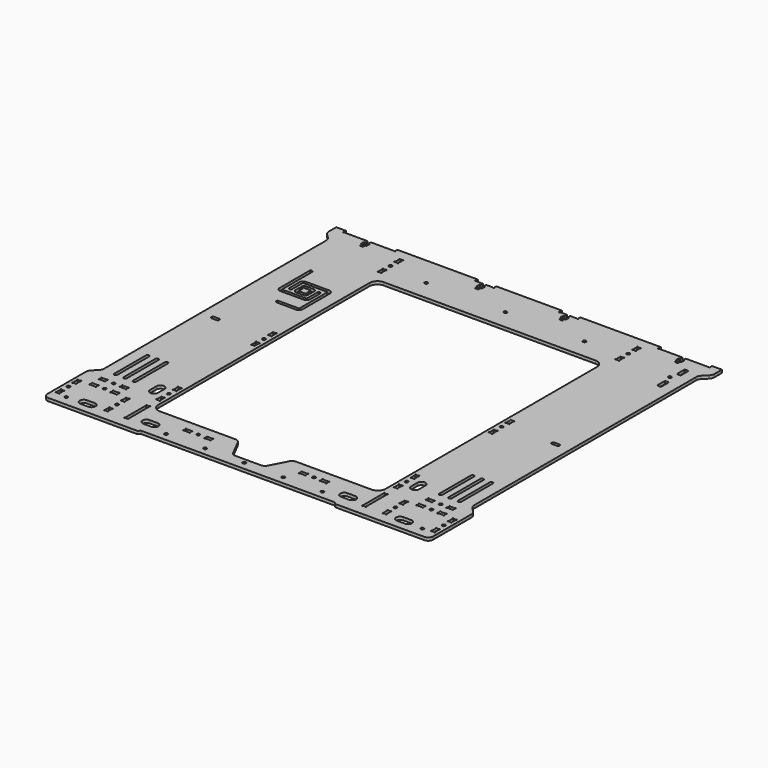
from build123d import *

# Parameters (mm, degrees)
F0_R     = 1.6
F1_DEPTH = 3


# Not quite as in the source:
# - ends of sketch curves that miss each other by under 0.0002 mm in the source are joined


with BuildPart() as f1:
    # F0 (on Top) → F1 (new body)
    with BuildSketch(Plane.XY):
        with BuildLine():
            Line((100.414611, -181.152447), (189.999995, -181.152721))
            ThreePointArc((189.999995, -181.152721), (193.5355256737, -179.6882531382), (194.99999, -176.152721))
            Line((194.99999, -176.152721), (194.99999, -127.617048))
            ThreePointArc((194.99999, -127.617048), (194.5500896571, -125.3374879994), (193.2678587346, -123.3997862741))
            Line((193.2678587346, -123.3997862741), (188.732131, -118.809631))
            ThreePointArc((188.732131, -118.809631), (187.4499003445, -116.8719290045), (187, -114.592369))
            Line((187, -114.592369), (187, 166.362005))
            ThreePointArc((187, 166.362005), (187.4567226696, 168.6581052675), (188.7573588129, 170.6046451871))
            Line((188.7573588129, 170.6046451871), (193.242641, 175.089927))
            ThreePointArc((193.242641, 175.089927), (194.5432773304, 177.0364667325), (195, 179.332567))
            Line((195, 179.332567), (195, 188.847286))
            Line((195, 188.847286), (185, 188.84728))
            Line((185, 188.84728), (185, 186.61326))
            ThreePointArc((185, 186.61326), (185.0669869604, 186.363259585), (185.2499996961, 186.1802464736))
            ThreePointArc((185.2499996961, 186.1802464736), (185.3535528736, 185.3936810924), (184.5669873396, 185.4972321961))
            ThreePointArc((184.5669873396, 185.4972321961), (184.3839752565, 185.6802441311), (184.133976, 185.747231))
            Line((184.133976, 185.747231), (160.775004, 185.747234))
            Line((160.775004, 185.747234), (160.775004, 182.747263))
            Line((160.775004, 182.747263), (162.049999, 182.747263))
            Line((162.049999, 182.747263), (162.049999, 178.747234))
            Line((162.049999, 178.747234), (160.775004, 178.747234))
            Line((160.775004, 178.747234), (160.775004, 175.747234))
            Line((160.775004, 175.747234), (157.574993, 175.747234))
            Line((157.574993, 175.747234), (157.574993, 178.747234))
            Line((157.574993, 178.747234), (156.299999, 178.747234))
            Line((156.299999, 178.747234), (156.299999, 182.747263))
            Line((156.299999, 182.747263), (157.574993, 182.747263))
            Line((157.574993, 182.747263), (157.574993, 185.747234))
            Line((157.574993, 185.747234), (134.066026, 185.74684))
            ThreePointArc((134.066026, 185.74684), (133.816025585, 185.6798530396), (133.6330124736, 185.4968403039))
            ThreePointArc((133.6330124736, 185.4968403039), (132.8464473986, 185.3932858203), (132.9499981961, 186.1798516604))
            ThreePointArc((132.9499981961, 186.1798516604), (133.1330100061, 186.362864527), (133.199997, 186.612864))
            Line((133.199997, 186.612864), (133.2, 188.846886))
            Line((133.2, 188.846886), (51.734412, 188.846886))
            Line((51.734412, 188.846886), (51.734412, 186.61287))
            ThreePointArc((51.734412, 186.61287), (51.8013990854, 186.3628693685), (51.9844121291, 186.1798562236))
            ThreePointArc((51.9844121291, 186.1798562236), (52.087966003, 185.3932912218), (51.3014003396, 185.4968421961))
            ThreePointArc((51.3014003396, 185.4968421961), (51.118387473, 185.6798540061), (50.868388, 185.746841))
            Line((50.868388, 185.746841), (44.100912, 185.74689))
            Line((44.100912, 185.74689), (44.100912, 182.74789))
            Line((44.100912, 182.74789), (45.375891, 182.747969))
            Line((45.375891, 182.747969), (45.375891, 178.747941))
            Line((45.375891, 178.747941), (44.100896, 178.747941))
            Line((44.100896, 178.747941), (44.100896, 175.747941))
            Line((44.100896, 175.747941), (40.900885, 175.747941))
            Line((40.900885, 175.747941), (40.900885, 178.747941))
            Line((40.900885, 178.747941), (39.625891, 178.747941))
            Line((39.625891, 178.747941), (39.625891, 182.747969))
            Line((39.625891, 182.747969), (40.900912, 182.74689))
            Line((40.900912, 182.74689), (40.900912, 185.74789))
            Line((40.900912, 185.74789), (34.131638, 185.746844))
            ThreePointArc((34.131638, 185.746844), (33.8816379355, 185.6798566646), (33.6986252236, 185.4968438709))
            ThreePointArc((33.6986252236, 185.4968438709), (32.9120602218, 185.393289997), (33.0156111961, 186.1798556604))
            ThreePointArc((33.0156111961, 186.1798556604), (33.1986222226, 186.362868902), (33.265609, 186.612868))
            Line((33.265609, 186.612868), (33.265612, 188.84689))
            Line((33.265612, 188.84689), (-33.265588, 188.84689))
            Line((-33.265588, 188.84689), (-33.265588, 186.61287))
            ThreePointArc((-33.265588, 186.61287), (-33.1986009146, 186.3628693685), (-33.0155878709, 186.1798562236))
            ThreePointArc((-33.0155878709, 186.1798562236), (-32.912033997, 185.3932912218), (-33.6985996604, 185.4968421961))
            ThreePointArc((-33.6985996604, 185.4968421961), (-33.881612527, 185.6798540061), (-34.131612, 185.746841))
            Line((-34.131612, 185.746841), (-40.908088, 185.74689))
            Line((-40.908088, 185.74689), (-40.908088, 182.74889))
            Line((-40.908088, 182.74889), (-39.633265, 182.748947))
            Line((-39.633265, 182.748947), (-39.633265, 178.748919))
            Line((-39.633265, 178.748919), (-40.90826, 178.748919))
            Line((-40.90826, 178.748919), (-40.90826, 175.748919))
            Line((-40.90826, 175.748919), (-44.108271, 175.748919))
            Line((-44.108271, 175.748919), (-44.108271, 178.748919))
            Line((-44.108271, 178.748919), (-45.383265, 178.748919))
            Line((-45.383265, 178.748919), (-45.383265, 182.748947))
            Line((-45.383265, 182.748947), (-44.108088, 182.74689))
            Line((-44.108088, 182.74689), (-44.108088, 185.74889))
            Line((-44.108088, 185.74889), (-50.876962, 185.746844))
            ThreePointArc((-50.876962, 185.746844), (-51.1269620645, 185.6798566646), (-51.3099747764, 185.4968438709))
            ThreePointArc((-51.3099747764, 185.4968438709), (-52.0965397782, 185.393289997), (-51.9929888039, 186.1798556604))
            ThreePointArc((-51.9929888039, 186.1798556604), (-51.8099777774, 186.362868902), (-51.742991, 186.612868))
            Line((-51.742991, 186.612868), (-51.742988, 188.846886))
            Line((-51.742988, 188.846886), (-133.2, 188.846886))
            Line((-133.2, 188.846886), (-133.2, 186.612866))
            ThreePointArc((-133.2, 186.612866), (-133.1330130396, 186.362865585), (-132.9500003039, 186.1798524736))
            ThreePointArc((-132.9500003039, 186.1798524736), (-132.8464458203, 185.3932873986), (-133.6330116604, 185.4968381961))
            ThreePointArc((-133.6330116604, 185.4968381961), (-133.816024527, 185.6798500061), (-134.066024, 185.746837))
            Line((-134.066024, 185.746837), (-157.574998, 185.747234))
            Line((-157.574998, 185.747234), (-157.574998, 182.747263))
            Line((-157.574998, 182.747263), (-156.300004, 182.747263))
            Line((-156.300004, 182.747263), (-156.300004, 178.747234))
            Line((-156.300004, 178.747234), (-157.574998, 178.747234))
            Line((-157.574998, 178.747234), (-157.574998, 175.747234))
            Line((-157.574998, 175.747234), (-160.775009, 175.747234))
            Line((-160.775009, 175.747234), (-160.775009, 178.747234))
            Line((-160.775009, 178.747234), (-162.050004, 178.747234))
            Line((-162.050004, 178.747234), (-162.050004, 182.747263))
            Line((-162.050004, 182.747263), (-160.775009, 182.747263))
            Line((-160.775009, 182.747263), (-160.775009, 185.747234))
            Line((-160.775009, 185.747234), (-184.133979, 185.747234))
            ThreePointArc((-184.133979, 185.747234), (-184.3839796315, 185.6802469146), (-184.5669927764, 185.4972338709))
            ThreePointArc((-184.5669927764, 185.4972338709), (-185.3535577782, 185.393679997), (-185.2500068039, 186.1802456604))
            ThreePointArc((-185.2500068039, 186.1802456604), (-185.0669949939, 186.363258527), (-185.000008, 186.613258))
            Line((-185.000008, 186.613258), (-185.000005, 188.84728))
            Line((-185.000005, 188.84728), (-195, 188.847286))
            Line((-195, 188.847286), (-195, 179.332567))
            ThreePointArc((-195, 179.332567), (-194.5432773304, 177.0364667325), (-193.2426411871, 175.0899268129))
            Line((-193.2426411871, 175.0899268129), (-188.757359, 170.604645))
            ThreePointArc((-188.757359, 170.604645), (-187.4567226696, 168.6581052675), (-187, 166.362005))
            Line((-187, 166.362005), (-187, -114.667433))
            ThreePointArc((-187, -114.667433), (-187.4567226696, -116.9635332675), (-188.7573588129, -118.9100731871))
            Line((-188.7573588129, -118.9100731871), (-193.242636, -123.39535))
            ThreePointArc((-193.242636, -123.39535), (-194.5432721951, -125.3418904058), (-194.999995, -127.637991))
            Line((-194.999995, -127.637991), (-194.999995, -176.152721))
            ThreePointArc((-194.999995, -176.152721), (-193.5355302491, -179.6882506633), (-190, -181.152714))
            Line((-190, -181.152714), (-100.41422, -181.152447))
            ThreePointArc((-100.41422, -181.152447), (-100.0315385085, -181.0763260938), (-99.7071167188, -180.8595542812))
            Line((-99.7071167188, -180.8595542812), (-98.292898, -179.445338))
            ThreePointArc((-98.292898, -179.445338), (-97.9684741057, -179.2285663322), (-97.585791, -179.152446))
            Line((-97.585791, -179.152446), (97.586183, -179.152446))
            ThreePointArc((97.586183, -179.152446), (97.9688657791, -179.2285661969), (98.2932887812, -179.4453382188))
            Line((98.2932887812, -179.4453382188), (99.707508, -180.859554))
            ThreePointArc((99.707508, -180.859554), (100.0319295085, -181.0763260938), (100.414611, -181.152447))
        make_face()
        with Locations((-180, -171.152714)):
            Circle(F0_R, mode=Mode.SUBTRACT)
        with BuildLine():
            Line((-190.603935, -163.652718), (-189.036068, -163.652721))
            ThreePointArc((-189.036068, -163.652721), (-188.7860679355, -163.5857336646), (-188.6030552236, -163.4027208709))
            ThreePointArc((-188.6030552236, -163.4027208709), (-187.8164902218, -163.299166997), (-187.9200411961, -164.0857326604))
            ThreePointArc((-187.9200411961, -164.0857326604), (-188.1030522226, -164.268745902), (-188.170039, -164.518745))
            Line((-188.170039, -164.518745), (-188.170039, -168.986694))
            ThreePointArc((-188.170039, -168.986694), (-188.1030520396, -169.236694415), (-187.9200393039, -169.4197075264))
            ThreePointArc((-187.9200393039, -169.4197075264), (-187.8164861264, -170.2062729076), (-188.6030516604, -170.1027218039))
            ThreePointArc((-188.6030516604, -170.1027218039), (-188.7860637435, -169.9197098689), (-189.036063, -169.852723))
            Line((-189.036063, -169.852723), (-190.603933, -169.85272))
            ThreePointArc((-190.603933, -169.85272), (-190.8539336315, -169.9197070854), (-191.0369467764, -170.1027201291))
            ThreePointArc((-191.0369467764, -170.1027201291), (-191.8235117782, -170.206274003), (-191.7199608039, -169.4197083396))
            ThreePointArc((-191.7199608039, -169.4197083396), (-191.5369489939, -169.236695473), (-191.469962, -168.986696))
            Line((-191.469962, -168.986696), (-191.469959, -164.518746))
            ThreePointArc((-191.469959, -164.518746), (-191.5369462104, -164.268746152), (-191.7199586961, -164.0857334736))
            ThreePointArc((-191.7199586961, -164.0857334736), (-191.8235131797, -163.2991683986), (-191.0369473396, -163.4027191961))
            ThreePointArc((-191.0369473396, -163.4027191961), (-190.853934473, -163.5857310061), (-190.603935, -163.652718))
        make_face(mode=Mode.SUBTRACT)
        with BuildLine():
            Line((-164.000002, -165.15272), (-156.000001, -165.15272))
            ThreePointArc((-156.000001, -165.15272), (-152.000001, -169.15272), (-156.000001, -173.15272))
            Line((-156.000001, -173.15272), (-164.000002, -173.152721))
            ThreePointArc((-164.000002, -173.152721), (-168.000002, -169.15272), (-164.000002, -165.15272))
        make_face(mode=Mode.SUBTRACT)
        with Locations((-189.820001, -156.152721)):
            Circle(F0_R, mode=Mode.SUBTRACT)
        with BuildLine():
            Line((-190.603935, -142.452719), (-189.036068, -142.452722))
            ThreePointArc((-189.036068, -142.452722), (-188.7860679355, -142.3857346646), (-188.6030552236, -142.2027218709))
            ThreePointArc((-188.6030552236, -142.2027218709), (-187.8164893986, -142.0991668203), (-187.9200409461, -142.8857330934))
            ThreePointArc((-187.9200409461, -142.8857330934), (-188.1030522226, -143.068745902), (-188.170039, -143.318745))
            Line((-188.170039, -143.318745), (-188.170039, -147.786695))
            ThreePointArc((-188.170039, -147.786695), (-188.1030517896, -148.036694848), (-187.9200393039, -148.2197075264))
            ThreePointArc((-187.9200393039, -148.2197075264), (-187.8164861264, -149.0062729076), (-188.6030516604, -148.9027218039))
            ThreePointArc((-188.6030516604, -148.9027218039), (-188.7860637435, -148.7197098689), (-189.036063, -148.652723))
            Line((-189.036063, -148.652723), (-190.603933, -148.65272))
            ThreePointArc((-190.603933, -148.65272), (-190.8539336315, -148.7197070854), (-191.0369467764, -148.9027201291))
            ThreePointArc((-191.0369467764, -148.9027201291), (-191.8235126014, -149.0062751797), (-191.7199610539, -148.2197089066))
            ThreePointArc((-191.7199610539, -148.2197089066), (-191.5369489939, -148.036696473), (-191.469962, -147.786697))
            Line((-191.469962, -147.786697), (-191.469959, -143.318747))
            ThreePointArc((-191.469959, -143.318747), (-191.5369462104, -143.068747152), (-191.7199586961, -142.8857344736))
            ThreePointArc((-191.7199586961, -142.8857344736), (-191.8235131797, -142.0991693986), (-191.0369473396, -142.2027201961))
            ThreePointArc((-191.0369473396, -142.2027201961), (-190.853934473, -142.3857320061), (-190.603935, -142.452719))
        make_face(mode=Mode.SUBTRACT)
        with BuildLine():
            Line((-179.000003, -141.936648), (-179, -140.368781))
            ThreePointArc((-179, -140.368781), (-179.0669872104, -140.118781152), (-179.2499996961, -139.9357684736))
            ThreePointArc((-179.2499996961, -139.9357684736), (-179.3535541797, -139.1492033986), (-178.5669883396, -139.2527541961))
            ThreePointArc((-178.5669883396, -139.2527541961), (-178.383975473, -139.4357660061), (-178.133976, -139.502753))
            Line((-178.133976, -139.502753), (-173.666026, -139.502753))
            ThreePointArc((-173.666026, -139.502753), (-173.416026152, -139.4357657896), (-173.2330134736, -139.2527533039))
            ThreePointArc((-173.2330134736, -139.2527533039), (-172.4464475753, -139.1491976435), (-172.5499989461, -139.9357640934))
            ThreePointArc((-172.5499989461, -139.9357640934), (-172.7330110061, -140.118776527), (-172.799998, -140.368776))
            Line((-172.799998, -140.368776), (-172.800001, -141.936647))
            ThreePointArc((-172.800001, -141.936647), (-172.7330137896, -142.186646848), (-172.5500013039, -142.3696595264))
            ThreePointArc((-172.5500013039, -142.3696595264), (-172.4464456435, -143.1562254247), (-173.2330120934, -143.0526740539))
            ThreePointArc((-173.2330120934, -143.0526740539), (-173.416024527, -142.8696619939), (-173.666024, -142.802675))
            Line((-173.666024, -142.802675), (-178.133974, -142.802672))
            ThreePointArc((-178.133974, -142.802672), (-178.383974415, -142.8696589604), (-178.5669875264, -143.0526716961))
            ThreePointArc((-178.5669875264, -143.0526716961), (-179.3535526014, -143.1562261797), (-179.2500018039, -142.3696603396))
            ThreePointArc((-179.2500018039, -142.3696603396), (-179.0669899939, -142.186647473), (-179.000003, -141.936648))
        make_face(mode=Mode.SUBTRACT)
        with Locations((-165.3, -141.152714)):
            Circle(F0_R, mode=Mode.SUBTRACT)
        with BuildLine():
            Line((-157.800003, -141.936648), (-157.8, -140.368781))
            ThreePointArc((-157.8, -140.368781), (-157.8669872104, -140.118781152), (-158.0499996961, -139.9357684736))
            ThreePointArc((-158.0499996961, -139.9357684736), (-158.1535553565, -139.1492025753), (-157.3669889066, -139.2527539461))
            ThreePointArc((-157.3669889066, -139.2527539461), (-157.183976473, -139.4357660061), (-156.933977, -139.502753))
            Line((-156.933977, -139.502753), (-152.466027, -139.502753))
            ThreePointArc((-152.466027, -139.502753), (-152.216026585, -139.4357660396), (-152.0330134736, -139.2527533039))
            ThreePointArc((-152.0330134736, -139.2527533039), (-151.2464475753, -139.1491976435), (-151.3499989461, -139.9357640934))
            ThreePointArc((-151.3499989461, -139.9357640934), (-151.5330110061, -140.118776527), (-151.599998, -140.368776))
            Line((-151.599998, -140.368776), (-151.600001, -141.936647))
            ThreePointArc((-151.600001, -141.936647), (-151.5330137896, -142.186646848), (-151.3500013039, -142.3696595264))
            ThreePointArc((-151.3500013039, -142.3696595264), (-151.2464468203, -143.1562246014), (-152.0330126604, -143.0526738039))
            ThreePointArc((-152.0330126604, -143.0526738039), (-152.216025527, -142.8696619939), (-152.466025, -142.802675))
            Line((-152.466025, -142.802675), (-156.933975, -142.802672))
            ThreePointArc((-156.933975, -142.802672), (-157.183974848, -142.8696592104), (-157.3669875264, -143.0526716961))
            ThreePointArc((-157.3669875264, -143.0526716961), (-158.1535526014, -143.1562261797), (-158.0500018039, -142.3696603396))
            ThreePointArc((-158.0500018039, -142.3696603396), (-157.8669899939, -142.186647473), (-157.800003, -141.936648))
        make_face(mode=Mode.SUBTRACT)
        with BuildLine():
            Line((-141.563935, -163.652718), (-139.996068, -163.652721))
            ThreePointArc((-139.996068, -163.652721), (-139.7460679355, -163.5857336646), (-139.5630552236, -163.4027208709))
            ThreePointArc((-139.5630552236, -163.4027208709), (-138.7764902218, -163.299166997), (-138.8800411961, -164.0857326604))
            ThreePointArc((-138.8800411961, -164.0857326604), (-139.0630522226, -164.268745902), (-139.130039, -164.518745))
            Line((-139.130039, -164.518745), (-139.130039, -168.986694))
            ThreePointArc((-139.130039, -168.986694), (-139.0630520396, -169.236694415), (-138.8800393039, -169.4197075264))
            ThreePointArc((-138.8800393039, -169.4197075264), (-138.7764861264, -170.2062729076), (-139.5630516604, -170.1027218039))
            ThreePointArc((-139.5630516604, -170.1027218039), (-139.7460637435, -169.9197098689), (-139.996063, -169.852723))
            Line((-139.996063, -169.852723), (-141.563933, -169.85272))
            ThreePointArc((-141.563933, -169.85272), (-141.8139336315, -169.9197070854), (-141.9969467764, -170.1027201291))
            ThreePointArc((-141.9969467764, -170.1027201291), (-142.7835117782, -170.206274003), (-142.6799608039, -169.4197083396))
            ThreePointArc((-142.6799608039, -169.4197083396), (-142.4969489939, -169.236695473), (-142.429962, -168.986696))
            Line((-142.429962, -168.986696), (-142.429959, -164.518746))
            ThreePointArc((-142.429959, -164.518746), (-142.4969462104, -164.268746152), (-142.6799586961, -164.0857334736))
            ThreePointArc((-142.6799586961, -164.0857334736), (-142.7835131797, -163.2991683986), (-141.9969473396, -163.4027191961))
            ThreePointArc((-141.9969473396, -163.4027191961), (-141.813934473, -163.5857310061), (-141.563935, -163.652718))
        make_face(mode=Mode.SUBTRACT)
        with BuildLine():
            Line((-104.000004, -160.752745), (-96.000003, -160.752745))
            ThreePointArc((-96.000003, -160.752745), (-92.000002, -164.752745), (-96.000003, -168.752746))
            Line((-96.000003, -168.752746), (-104.000004, -168.752746))
            ThreePointArc((-104.000004, -168.752746), (-108.000005, -164.752745), (-104.000004, -160.752745))
        make_face(mode=Mode.SUBTRACT)
        with Locations((-140.78, -156.152721)):
            Circle(F0_R, mode=Mode.SUBTRACT)
        with BuildLine():
            Line((-141.563935, -142.452719), (-139.996068, -142.452722))
            ThreePointArc((-139.996068, -142.452722), (-139.7460679355, -142.3857346646), (-139.5630552236, -142.2027218709))
            ThreePointArc((-139.5630552236, -142.2027218709), (-138.7764893986, -142.0991668203), (-138.8800409461, -142.8857330934))
            ThreePointArc((-138.8800409461, -142.8857330934), (-139.0630522226, -143.068745902), (-139.130039, -143.318745))
            Line((-139.130039, -143.318745), (-139.130039, -147.786695))
            ThreePointArc((-139.130039, -147.786695), (-139.0630517896, -148.036694848), (-138.8800393039, -148.2197075264))
            ThreePointArc((-138.8800393039, -148.2197075264), (-138.7764861264, -149.0062729076), (-139.5630516604, -148.9027218039))
            ThreePointArc((-139.5630516604, -148.9027218039), (-139.7460637435, -148.7197098689), (-139.996063, -148.652723))
            Line((-139.996063, -148.652723), (-141.563933, -148.65272))
            ThreePointArc((-141.563933, -148.65272), (-141.8139336315, -148.7197070854), (-141.9969467764, -148.9027201291))
            ThreePointArc((-141.9969467764, -148.9027201291), (-142.7835126014, -149.0062751797), (-142.6799610539, -148.2197089066))
            ThreePointArc((-142.6799610539, -148.2197089066), (-142.4969489939, -148.036696473), (-142.429962, -147.786697))
            Line((-142.429962, -147.786697), (-142.429959, -143.318747))
            ThreePointArc((-142.429959, -143.318747), (-142.4969462104, -143.068747152), (-142.6799586961, -142.8857344736))
            ThreePointArc((-142.6799586961, -142.8857344736), (-142.7835131797, -142.0991693986), (-141.9969473396, -142.2027201961))
            ThreePointArc((-141.9969473396, -142.2027201961), (-141.813934473, -142.3857320061), (-141.563935, -142.452719))
        make_face(mode=Mode.SUBTRACT)
        with BuildLine():
            Line((-120.958936, -142.452719), (-119.391069, -142.452722))
            ThreePointArc((-119.391069, -142.452722), (-119.1410695024, -142.3857344146), (-118.9580572236, -142.2027218709))
            ThreePointArc((-118.9580572236, -142.2027218709), (-118.1714913986, -142.0991668203), (-118.2750429461, -142.8857330934))
            ThreePointArc((-118.2750429461, -142.8857330934), (-118.4580542226, -143.068745902), (-118.525041, -143.318745))
            Line((-118.525041, -143.318745), (-118.525041, -168.986694))
            ThreePointArc((-118.525041, -168.986694), (-118.4580540396, -169.236694415), (-118.2750413039, -169.4197075264))
            ThreePointArc((-118.2750413039, -169.4197075264), (-118.1714858203, -170.2062736014), (-118.9580523434, -170.1027216209))
            ThreePointArc((-118.9580523434, -170.1027216209), (-119.1410647435, -169.9197098689), (-119.391064, -169.852723))
            Line((-119.391064, -169.852723), (-120.958935, -169.85272))
            ThreePointArc((-120.958935, -169.85272), (-121.2089350645, -169.9197073354), (-121.3919477764, -170.1027201291))
            ThreePointArc((-121.3919477764, -170.1027201291), (-122.1785127782, -170.206274003), (-122.0749618039, -169.4197083396))
            ThreePointArc((-122.0749618039, -169.4197083396), (-121.8919499939, -169.236695473), (-121.824963, -168.986696))
            Line((-121.824963, -168.986696), (-121.82496, -143.318747))
            ThreePointArc((-121.82496, -143.318747), (-121.8919472104, -143.068747152), (-122.0749596961, -142.8857344736))
            ThreePointArc((-122.0749596961, -142.8857344736), (-122.1785141797, -142.0991693986), (-121.3919483396, -142.2027201961))
            ThreePointArc((-121.3919483396, -142.2027201961), (-121.208935473, -142.3857320061), (-120.958936, -142.452719))
        make_face(mode=Mode.SUBTRACT)
        with BuildLine():
            Line((-179.000011, -130.291654), (-179.000008, -128.723787))
            ThreePointArc((-179.000008, -128.723787), (-179.0669952104, -128.473787152), (-179.2500076961, -128.2907744736))
            ThreePointArc((-179.2500076961, -128.2907744736), (-179.3535621797, -127.5042093986), (-178.5669963396, -127.6077601961))
            ThreePointArc((-178.5669963396, -127.6077601961), (-178.383983473, -127.7907720061), (-178.133984, -127.857759))
            Line((-178.133984, -127.857759), (-173.666034, -127.857759))
            ThreePointArc((-173.666034, -127.857759), (-173.4160345024, -127.7907714146), (-173.2330222236, -127.6077588709))
            ThreePointArc((-173.2330222236, -127.6077588709), (-172.4464563986, -127.5042038203), (-172.5500079461, -128.2907700934))
            ThreePointArc((-172.5500079461, -128.2907700934), (-172.7330192226, -128.473782902), (-172.800006, -128.723782))
            Line((-172.800006, -128.723782), (-172.800009, -130.291653))
            ThreePointArc((-172.800009, -130.291653), (-172.7330217896, -130.541652848), (-172.5500093039, -130.7246655264))
            ThreePointArc((-172.5500093039, -130.7246655264), (-172.4464538203, -131.5112316014), (-173.2330203434, -131.4076796209))
            ThreePointArc((-173.2330203434, -131.4076796209), (-173.4160327435, -131.2246678689), (-173.666032, -131.157681))
            Line((-173.666032, -131.157681), (-178.133982, -131.157678))
            ThreePointArc((-178.133982, -131.157678), (-178.3839826315, -131.2246650854), (-178.5669957764, -131.4076781291))
            ThreePointArc((-178.5669957764, -131.4076781291), (-179.3535607782, -131.511232003), (-179.2500098039, -130.7246663396))
            ThreePointArc((-179.2500098039, -130.7246663396), (-179.0669979939, -130.541653473), (-179.000011, -130.291654))
        make_face(mode=Mode.SUBTRACT)
        with Locations((-165.300008, -129.50772)):
            Circle(F0_R, mode=Mode.SUBTRACT)
        with BuildLine():
            Line((-157.800011, -130.291654), (-157.800008, -128.723787))
            ThreePointArc((-157.800008, -128.723787), (-157.8669952104, -128.473787152), (-158.0500076961, -128.2907744736))
            ThreePointArc((-158.0500076961, -128.2907744736), (-158.1535633565, -127.5042085753), (-157.3669969066, -127.6077599461))
            ThreePointArc((-157.3669969066, -127.6077599461), (-157.183984473, -127.7907720061), (-156.933985, -127.857759))
            Line((-156.933985, -127.857759), (-152.466035, -127.857759))
            ThreePointArc((-152.466035, -127.857759), (-152.2160349355, -127.7907716646), (-152.0330222236, -127.6077588709))
            ThreePointArc((-152.0330222236, -127.6077588709), (-151.2464563986, -127.5042038203), (-151.3500079461, -128.2907700934))
            ThreePointArc((-151.3500079461, -128.2907700934), (-151.5330192226, -128.473782902), (-151.600006, -128.723782))
            Line((-151.600006, -128.723782), (-151.600009, -130.291653))
            ThreePointArc((-151.600009, -130.291653), (-151.5330217896, -130.541652848), (-151.3500093039, -130.7246655264))
            ThreePointArc((-151.3500093039, -130.7246655264), (-151.2464561264, -131.5112309076), (-152.0330216604, -131.4076798039))
            ThreePointArc((-152.0330216604, -131.4076798039), (-152.2160337435, -131.2246678689), (-152.466033, -131.157681))
            Line((-152.466033, -131.157681), (-156.933983, -131.157678))
            ThreePointArc((-156.933983, -131.157678), (-157.1839830645, -131.2246653354), (-157.3669957764, -131.4076781291))
            ThreePointArc((-157.3669957764, -131.4076781291), (-158.1535607782, -131.511232003), (-158.0500098039, -130.7246663396))
            ThreePointArc((-158.0500098039, -130.7246663396), (-157.8669979939, -130.541653473), (-157.800011, -130.291654))
        make_face(mode=Mode.SUBTRACT)
        with BuildLine():
            Line((-175.4, -116.152714), (-175.4, -76.152714))
            ThreePointArc((-175.4, -76.152714), (-173.8, -74.552714), (-172.2, -76.152714))
            Line((-172.2, -76.152714), (-172.2, -116.152714))
            ThreePointArc((-172.2, -116.152714), (-173.8, -117.752714), (-175.4, -116.152714))
        make_face(mode=Mode.SUBTRACT)
        with BuildLine():
            Line((-165.9, -116.152714), (-165.9, -76.152714))
            ThreePointArc((-165.9, -76.152714), (-164.3, -74.552714), (-162.7, -76.152714))
            Line((-162.7, -76.152714), (-162.7, -116.152714))
            ThreePointArc((-162.7, -116.152714), (-164.3, -117.752714), (-165.9, -116.152714))
        make_face(mode=Mode.SUBTRACT)
        with BuildLine():
            Line((-156.4, -116.152714), (-156.4, -76.152714))
            ThreePointArc((-156.4, -76.152714), (-154.8, -74.552714), (-153.2, -76.152714))
            Line((-153.2, -76.152714), (-153.2, -116.152714))
            ThreePointArc((-153.2, -116.152714), (-154.8, -117.752714), (-156.4, -116.152714))
        make_face(mode=Mode.SUBTRACT)
        with BuildLine():
            Line((-128.000001, -112.152716), (-128.000001, -120.152716))
            ThreePointArc((-128.000001, -120.152716), (-132.0000005, -124.152716), (-136.000001, -120.152717))
            Line((-136.000001, -120.152717), (-136.000001, -112.152717))
            ThreePointArc((-136.000001, -112.152717), (-132.0000015, -108.152716), (-128.000001, -112.152716))
        make_face(mode=Mode.SUBTRACT)
        with BuildLine():
            Line((-121.824919, -128.986627), (-121.824919, -124.518677))
            ThreePointArc((-121.824919, -124.518677), (-121.8919059939, -124.268677527), (-122.0749179461, -124.0856649066))
            ThreePointArc((-122.0749179461, -124.0856649066), (-122.1784687782, -123.299098997), (-121.3919034736, -123.4026526961))
            ThreePointArc((-121.3919034736, -123.4026526961), (-121.2088910645, -123.5856656646), (-120.958891, -123.652653))
            Line((-120.958891, -123.652653), (-119.391023, -123.65265))
            ThreePointArc((-119.391023, -123.65265), (-119.1410237435, -123.5856631311), (-118.9580111566, -123.4026514869))
            ThreePointArc((-118.9580111566, -123.4026514869), (-118.1714448203, -123.2990993986), (-118.2750003121, -124.0856654594))
            ThreePointArc((-118.2750003121, -124.0856654594), (-118.4580130396, -124.268678585), (-118.525, -124.518679))
            Line((-118.525, -124.518679), (-118.524997, -128.986629))
            ThreePointArc((-118.524997, -128.986629), (-118.4580102226, -129.236628098), (-118.2749988039, -129.4196406604))
            ThreePointArc((-118.2749988039, -129.4196406604), (-118.1714473986, -130.2062071797), (-118.9580132094, -130.1026521209))
            ThreePointArc((-118.9580132094, -130.1026521209), (-119.1410255024, -129.9196395854), (-119.391025, -129.852652))
            Line((-119.391025, -129.852652), (-120.958895, -129.852655))
            ThreePointArc((-120.958895, -129.852655), (-121.208894098, -129.9196417774), (-121.3919066604, -130.1026531961))
            ThreePointArc((-121.3919066604, -130.1026531961), (-122.1784728736, -130.2062049076), (-122.0749188709, -129.4196392236))
            ThreePointArc((-122.0749188709, -129.4196392236), (-121.8919062104, -129.236626848), (-121.824919, -128.986627))
        make_face(mode=Mode.SUBTRACT)
        with Locations((-120.174958, -116.152653)):
            Circle(F0_R, mode=Mode.SUBTRACT)
        with BuildLine():
            Line((-121.824919, -107.786627), (-121.824919, -103.318678))
            ThreePointArc((-121.824919, -103.318678), (-121.8919059939, -103.068678527), (-122.0749179461, -102.8856659066))
            ThreePointArc((-122.0749179461, -102.8856659066), (-122.1784687782, -102.099099997), (-121.3919034736, -102.2026536961))
            ThreePointArc((-121.3919034736, -102.2026536961), (-121.2088910645, -102.3856666646), (-120.958891, -102.452654))
            Line((-120.958891, -102.452654), (-119.391023, -102.452651))
            ThreePointArc((-119.391023, -102.452651), (-119.1410237435, -102.3856641311), (-118.9580111566, -102.2026524869))
            ThreePointArc((-118.9580111566, -102.2026524869), (-118.1714448203, -102.0991003986), (-118.2750003121, -102.8856664594))
            ThreePointArc((-118.2750003121, -102.8856664594), (-118.4580127896, -103.068679152), (-118.525, -103.318679))
            Line((-118.525, -103.318679), (-118.524997, -107.786629))
            ThreePointArc((-118.524997, -107.786629), (-118.4580102226, -108.036628098), (-118.2749988039, -108.2196406604))
            ThreePointArc((-118.2749988039, -108.2196406604), (-118.1714482218, -109.006207003), (-118.9580135264, -108.9026533039))
            ThreePointArc((-118.9580135264, -108.9026533039), (-119.1410255024, -108.7196405854), (-119.391025, -108.652653))
            Line((-119.391025, -108.652653), (-120.958895, -108.652656))
            ThreePointArc((-120.958895, -108.652656), (-121.208894473, -108.7196429939), (-121.3919070934, -108.9026549461))
            ThreePointArc((-121.3919070934, -108.9026549461), (-122.1784731797, -109.0062056014), (-122.0749188709, -108.2196402236))
            ThreePointArc((-122.0749188709, -108.2196402236), (-121.8919059604, -108.036627415), (-121.824919, -107.786627))
        make_face(mode=Mode.SUBTRACT)
        with Locations((-79.016604, -171.152746)):
            Circle(F0_R, mode=Mode.SUBTRACT)
        with BuildLine():
            Line((-72.225046, -156.936653), (-72.225043, -155.368786))
            ThreePointArc((-72.225043, -155.368786), (-72.2920305854, -155.1187865024), (-72.4750431291, -154.9357742236))
            ThreePointArc((-72.4750431291, -154.9357742236), (-72.5785958736, -154.1492090924), (-71.7920305896, -154.2527597631))
            ThreePointArc((-71.7920305896, -154.2527597631), (-71.609018098, -154.4357712226), (-71.359019, -154.502758))
            Line((-71.359019, -154.502758), (-66.891069, -154.502758))
            ThreePointArc((-66.891069, -154.502758), (-66.641069152, -154.4357707896), (-66.4580564736, -154.2527583039))
            ThreePointArc((-66.4580564736, -154.2527583039), (-65.6714903986, -154.1492028203), (-65.7750423791, -154.9357693434))
            ThreePointArc((-65.7750423791, -154.9357693434), (-65.9580541311, -155.1187817435), (-66.025041, -155.368781))
            Line((-66.025041, -155.368781), (-66.025044, -156.936652))
            ThreePointArc((-66.025044, -156.936652), (-65.9580566646, -157.1866520645), (-65.7750438709, -157.3696647764))
            ThreePointArc((-65.7750438709, -157.3696647764), (-65.6714888203, -158.1562306014), (-66.4580550934, -158.0526790539))
            ThreePointArc((-66.4580550934, -158.0526790539), (-66.641067527, -157.8696669939), (-66.891067, -157.80268))
            Line((-66.891067, -157.80268), (-71.359017, -157.802677))
            ThreePointArc((-71.359017, -157.802677), (-71.609017415, -157.8696639604), (-71.7920305264, -158.0526766961))
            ThreePointArc((-71.7920305264, -158.0526766961), (-72.5785959076, -158.1562308736), (-72.4750440539, -157.3696649066))
            ThreePointArc((-72.4750440539, -157.3696649066), (-72.2920327774, -157.186652098), (-72.225046, -156.936653))
        make_face(mode=Mode.SUBTRACT)
        with Locations((-58.525043, -156.152719)):
            Circle(F0_R, mode=Mode.SUBTRACT)
        with Locations((-39.508604, -171.152746)):
            Circle(F0_R, mode=Mode.SUBTRACT)
        with BuildLine():
            Line((-51.025046, -156.936653), (-51.025043, -155.368786))
            ThreePointArc((-51.025043, -155.368786), (-51.0920305854, -155.1187865024), (-51.2750431291, -154.9357742236))
            ThreePointArc((-51.2750431291, -154.9357742236), (-51.3785981797, -154.1492083986), (-50.5920319066, -154.2527599461))
            ThreePointArc((-50.5920319066, -154.2527599461), (-50.409019098, -154.4357712226), (-50.15902, -154.502758))
            Line((-50.15902, -154.502758), (-45.69107, -154.502758))
            ThreePointArc((-45.69107, -154.502758), (-45.441069585, -154.4357710396), (-45.2580564736, -154.2527583039))
            ThreePointArc((-45.2580564736, -154.2527583039), (-44.4714903986, -154.1492028203), (-44.5750423791, -154.9357693434))
            ThreePointArc((-44.5750423791, -154.9357693434), (-44.7580541311, -155.1187817435), (-44.825041, -155.368781))
            Line((-44.825041, -155.368781), (-44.825044, -156.936652))
            ThreePointArc((-44.825044, -156.936652), (-44.7580566646, -157.1866520645), (-44.5750438709, -157.3696647764))
            ThreePointArc((-44.5750438709, -157.3696647764), (-44.471489997, -158.1562297782), (-45.2580556604, -158.0526788039))
            ThreePointArc((-45.2580556604, -158.0526788039), (-45.441068527, -157.8696669939), (-45.691068, -157.80268))
            Line((-45.691068, -157.80268), (-50.159018, -157.802677))
            ThreePointArc((-50.159018, -157.802677), (-50.409017848, -157.8696642104), (-50.5920305264, -158.0526766961))
            ThreePointArc((-50.5920305264, -158.0526766961), (-51.3785959076, -158.1562308736), (-51.2750440539, -157.3696649066))
            ThreePointArc((-51.2750440539, -157.3696649066), (-51.0920327774, -157.186652098), (-51.025046, -156.936653))
        make_face(mode=Mode.SUBTRACT)
        with BuildLine():
            Line((-120.958936, -3.65271), (-119.391069, -3.652713))
            ThreePointArc((-119.391069, -3.652713), (-119.1410695024, -3.5857254146), (-118.9580572236, -3.4027128709))
            ThreePointArc((-118.9580572236, -3.4027128709), (-118.1714922218, -3.299158997), (-118.2750431961, -4.0857246604))
            ThreePointArc((-118.2750431961, -4.0857246604), (-118.4580542226, -4.268737902), (-118.525041, -4.518737))
            Line((-118.525041, -4.518737), (-118.525041, -8.986687))
            ThreePointArc((-118.525041, -8.986687), (-118.4580537896, -9.236686848), (-118.2750413039, -9.4196995264))
            ThreePointArc((-118.2750413039, -9.4196995264), (-118.1714858203, -10.2062656014), (-118.9580523434, -10.1027136209))
            ThreePointArc((-118.9580523434, -10.1027136209), (-119.1410647435, -9.9197018689), (-119.391064, -9.852715))
            Line((-119.391064, -9.852715), (-120.958935, -9.852712))
            ThreePointArc((-120.958935, -9.852712), (-121.2089350645, -9.9196993354), (-121.3919477764, -10.1027121291))
            ThreePointArc((-121.3919477764, -10.1027121291), (-122.1785136014, -10.2062671797), (-122.0749620539, -9.4197009066))
            ThreePointArc((-122.0749620539, -9.4197009066), (-121.8919499939, -9.236688473), (-121.824963, -8.986689))
            Line((-121.824963, -8.986689), (-121.82496, -4.518739))
            ThreePointArc((-121.82496, -4.518739), (-121.8919469604, -4.268738585), (-122.0749596961, -4.0857254736))
            ThreePointArc((-122.0749596961, -4.0857254736), (-122.1785141797, -3.2991603986), (-121.3919483396, -3.4027111961))
            ThreePointArc((-121.3919483396, -3.4027111961), (-121.208935473, -3.5857230061), (-120.958936, -3.65271))
        make_face(mode=Mode.SUBTRACT)
        with Locations((0, -171.152714)):
            Circle(F0_R, mode=Mode.SUBTRACT)
        with Locations((39.508396, -171.152746)):
            Circle(F0_R, mode=Mode.SUBTRACT)
        with BuildLine():
            Line((44.825036, -156.936674), (44.825039, -155.368807))
            ThreePointArc((44.825039, -155.368807), (44.7580514146, -155.1188075024), (44.5750388709, -154.9357952236))
            ThreePointArc((44.5750388709, -154.9357952236), (44.4714851264, -154.1492290924), (45.2580510934, -154.2527809461))
            ThreePointArc((45.2580510934, -154.2527809461), (45.441063902, -154.4357922226), (45.691063, -154.502779))
            Line((45.691063, -154.502779), (50.159013, -154.502779))
            ThreePointArc((50.159013, -154.502779), (50.4090124976, -154.4357914146), (50.5920247764, -154.2527788709))
            ThreePointArc((50.5920247764, -154.2527788709), (51.3785906014, -154.1492238203), (51.2750390539, -154.9357900934))
            ThreePointArc((51.2750390539, -154.9357900934), (51.0920277774, -155.118802902), (51.025041, -155.368802))
            Line((51.025041, -155.368802), (51.025038, -156.936673))
            ThreePointArc((51.025038, -156.936673), (51.0920252104, -157.186672848), (51.2750376961, -157.3696855264))
            ThreePointArc((51.2750376961, -157.3696855264), (51.3785933565, -158.1562514247), (50.5920269066, -158.0527000539))
            ThreePointArc((50.5920269066, -158.0527000539), (50.409014473, -157.8696879939), (50.159015, -157.802701))
            Line((50.159015, -157.802701), (45.691065, -157.802698))
            ThreePointArc((45.691065, -157.802698), (45.4410643685, -157.8696850854), (45.2580512236, -158.0526981291))
            ThreePointArc((45.2580512236, -158.0526981291), (44.4714862218, -158.156252003), (44.5750371961, -157.3696863396))
            ThreePointArc((44.5750371961, -157.3696863396), (44.7580490061, -157.186673473), (44.825036, -156.936674))
        make_face(mode=Mode.SUBTRACT)
        with Locations((79.016396, -171.152746)):
            Circle(F0_R, mode=Mode.SUBTRACT)
        with Locations((58.525039, -156.15274)):
            Circle(F0_R, mode=Mode.SUBTRACT)
        with BuildLine():
            Line((66.025036, -156.936674), (66.025039, -155.368807))
            ThreePointArc((66.025039, -155.368807), (65.9580514146, -155.1188075024), (65.7750388709, -154.9357952236))
            ThreePointArc((65.7750388709, -154.9357952236), (65.6714838203, -154.1492293986), (66.4580500934, -154.2527809461))
            ThreePointArc((66.4580500934, -154.2527809461), (66.641062902, -154.4357922226), (66.891062, -154.502779))
            Line((66.891062, -154.502779), (71.359012, -154.502779))
            ThreePointArc((71.359012, -154.502779), (71.6090120645, -154.4357916646), (71.7920247764, -154.2527788709))
            ThreePointArc((71.7920247764, -154.2527788709), (72.5785906014, -154.1492238203), (72.4750390539, -154.9357900934))
            ThreePointArc((72.4750390539, -154.9357900934), (72.2920277774, -155.118802902), (72.225041, -155.368802))
            Line((72.225041, -155.368802), (72.225038, -156.936673))
            ThreePointArc((72.225038, -156.936673), (72.2920252104, -157.186672848), (72.4750376961, -157.3696855264))
            ThreePointArc((72.4750376961, -157.3696855264), (72.5785910503, -158.1562507309), (71.7920255896, -158.0527002369))
            ThreePointArc((71.7920255896, -158.0527002369), (71.609013473, -157.8696879939), (71.359014, -157.802701))
            Line((71.359014, -157.802701), (66.891064, -157.802698))
            ThreePointArc((66.891064, -157.802698), (66.6410639355, -157.8696853354), (66.4580512236, -158.0526981291))
            ThreePointArc((66.4580512236, -158.0526981291), (65.6714862218, -158.156252003), (65.7750371961, -157.3696863396))
            ThreePointArc((65.7750371961, -157.3696863396), (65.9580490061, -157.186673473), (66.025036, -156.936674))
        make_face(mode=Mode.SUBTRACT)
        with BuildLine():
            Line((95.999994, -160.752745), (103.999995, -160.752745))
            ThreePointArc((103.999995, -160.752745), (107.999996, -164.752745), (103.999995, -168.752746))
            Line((103.999995, -168.752746), (95.999994, -168.752746))
            ThreePointArc((95.999994, -168.752746), (91.999993, -164.752745), (95.999994, -160.752745))
        make_face(mode=Mode.SUBTRACT)
        with BuildLine():
            Line((139.130079, -168.986624), (139.130079, -164.518674))
            ThreePointArc((139.130079, -164.518674), (139.0630920061, -164.268674527), (138.8800800539, -164.0856619066))
            ThreePointArc((138.8800800539, -164.0856619066), (138.7765283986, -163.2990958203), (139.5630942094, -163.4026508791))
            ThreePointArc((139.5630942094, -163.4026508791), (139.7461069355, -163.5856636646), (139.996107, -163.652651))
            Line((139.996107, -163.652651), (141.563975, -163.652648))
            ThreePointArc((141.563975, -163.652648), (141.8139742565, -163.5856611311), (141.9969868434, -163.4026494869))
            ThreePointArc((141.9969868434, -163.4026494869), (142.7835531797, -163.2990973986), (142.6799976879, -164.0856634594))
            ThreePointArc((142.6799976879, -164.0856634594), (142.4969852104, -164.268676152), (142.429998, -164.518676))
            Line((142.429998, -164.518676), (142.430001, -168.986626))
            ThreePointArc((142.430001, -168.986626), (142.4969877774, -169.236625098), (142.6799991961, -169.4196376604))
            ThreePointArc((142.6799991961, -169.4196376604), (142.7835506014, -170.2062041797), (141.9969847906, -170.1026491209))
            ThreePointArc((141.9969847906, -170.1026491209), (141.8139724976, -169.9196365854), (141.563973, -169.852649))
            Line((141.563973, -169.852649), (139.996103, -169.852652))
            ThreePointArc((139.996103, -169.852652), (139.746103527, -169.9196389939), (139.5630909066, -170.1026509461))
            ThreePointArc((139.5630909066, -170.1026509461), (138.7765248203, -170.2062016014), (138.8800791291, -169.4196362236))
            ThreePointArc((138.8800791291, -169.4196362236), (139.0630917896, -169.236623848), (139.130079, -168.986624))
        make_face(mode=Mode.SUBTRACT)
        with BuildLine():
            Line((119.391063, -142.452719), (120.95893, -142.452722))
            ThreePointArc((120.95893, -142.452722), (121.2089300645, -142.3857346646), (121.3919427764, -142.2027218709))
            ThreePointArc((121.3919427764, -142.2027218709), (122.1785086014, -142.0991668203), (122.0749570539, -142.8857330934))
            ThreePointArc((122.0749570539, -142.8857330934), (121.8919457774, -143.068745902), (121.824959, -143.318745))
            Line((121.824959, -143.318745), (121.824959, -168.986694))
            ThreePointArc((121.824959, -168.986694), (121.8919459604, -169.236694415), (122.0749586961, -169.4197075264))
            ThreePointArc((122.0749586961, -169.4197075264), (122.1785118736, -170.2062729076), (121.3919463396, -170.1027218039))
            ThreePointArc((121.3919463396, -170.1027218039), (121.2089342565, -169.9197098689), (120.958935, -169.852723))
            Line((120.958935, -169.852723), (119.391065, -169.85272))
            ThreePointArc((119.391065, -169.85272), (119.1410643685, -169.9197070854), (118.9580512236, -170.1027201291))
            ThreePointArc((118.9580512236, -170.1027201291), (118.1714862218, -170.206274003), (118.2750371961, -169.4197083396))
            ThreePointArc((118.2750371961, -169.4197083396), (118.4580490061, -169.236695473), (118.525036, -168.986696))
            Line((118.525036, -168.986696), (118.525039, -143.318747))
            ThreePointArc((118.525039, -143.318747), (118.4580517896, -143.068747152), (118.2750393039, -142.8857344736))
            ThreePointArc((118.2750393039, -142.8857344736), (118.1714848203, -142.0991693986), (118.9580506604, -142.2027201961))
            ThreePointArc((118.9580506604, -142.2027201961), (119.141063527, -142.3857320061), (119.391063, -142.452719))
        make_face(mode=Mode.SUBTRACT)
        with Locations((140.78004, -156.15265)):
            Circle(F0_R, mode=Mode.SUBTRACT)
        with BuildLine():
            Line((139.130079, -147.786625), (139.130079, -143.318675))
            ThreePointArc((139.130079, -143.318675), (139.0630920061, -143.068675527), (138.8800800539, -142.8856629066))
            ThreePointArc((138.8800800539, -142.8856629066), (138.7765292218, -142.099096997), (139.5630945264, -142.2026506961))
            ThreePointArc((139.5630945264, -142.2026506961), (139.7461069355, -142.3856636646), (139.996107, -142.452651))
            Line((139.996107, -142.452651), (141.563975, -142.452648))
            ThreePointArc((141.563975, -142.452648), (141.8139742565, -142.3856611311), (141.9969868434, -142.2026494869))
            ThreePointArc((141.9969868434, -142.2026494869), (142.7835531797, -142.0990973986), (142.6799976879, -142.8856634594))
            ThreePointArc((142.6799976879, -142.8856634594), (142.4969849604, -143.068676585), (142.429998, -143.318677))
            Line((142.429998, -143.318677), (142.430001, -147.786626))
            ThreePointArc((142.430001, -147.786626), (142.4969877774, -148.036625098), (142.6799991961, -148.2196376604))
            ThreePointArc((142.6799991961, -148.2196376604), (142.7835497782, -149.006204003), (141.9969844736, -148.9026503039))
            ThreePointArc((141.9969844736, -148.9026503039), (141.8139724976, -148.7196375854), (141.563973, -148.65265))
            Line((141.563973, -148.65265), (139.996103, -148.652653))
            ThreePointArc((139.996103, -148.652653), (139.746103902, -148.7196397774), (139.5630913396, -148.9026511961))
            ThreePointArc((139.5630913396, -148.9026511961), (138.7765251264, -149.0062029076), (138.8800791291, -148.2196372236))
            ThreePointArc((138.8800791291, -148.2196372236), (139.0630917896, -148.036624848), (139.130079, -147.786625))
        make_face(mode=Mode.SUBTRACT)
        with BuildLine():
            Line((164.000002, -173.152721), (156.000001, -173.152721))
            ThreePointArc((156.000001, -173.152721), (152.000001, -169.15272), (156.000001, -165.15272))
            Line((156.000001, -165.15272), (164.000002, -165.15272))
            ThreePointArc((164.000002, -165.15272), (168.000002, -169.15272), (164.000002, -173.152721))
        make_face(mode=Mode.SUBTRACT)
        with Locations((180, -171.152714)):
            Circle(F0_R, mode=Mode.SUBTRACT)
        with BuildLine():
            Line((188.170079, -168.986617), (188.170079, -164.518667))
            ThreePointArc((188.170079, -164.518667), (188.1030920061, -164.268667527), (187.9200800539, -164.0856549066))
            ThreePointArc((187.9200800539, -164.0856549066), (187.8165283986, -163.2990888203), (188.6030942094, -163.4026438791))
            ThreePointArc((188.6030942094, -163.4026438791), (188.7861069355, -163.5856566646), (189.036107, -163.652644))
            Line((189.036107, -163.652644), (190.603975, -163.652641))
            ThreePointArc((190.603975, -163.652641), (190.8539742565, -163.5856541311), (191.0369868434, -163.4026424869))
            ThreePointArc((191.0369868434, -163.4026424869), (191.8235531797, -163.2990903986), (191.7199976879, -164.0856564594))
            ThreePointArc((191.7199976879, -164.0856564594), (191.5369852104, -164.268669152), (191.469998, -164.518669))
            Line((191.469998, -164.518669), (191.470001, -168.986619))
            ThreePointArc((191.470001, -168.986619), (191.5369877774, -169.236618098), (191.7199991961, -169.4196306604))
            ThreePointArc((191.7199991961, -169.4196306604), (191.8235506014, -170.2061971797), (191.0369847906, -170.1026421209))
            ThreePointArc((191.0369847906, -170.1026421209), (190.8539724976, -169.9196295854), (190.603973, -169.852642))
            Line((190.603973, -169.852642), (189.036103, -169.852645))
            ThreePointArc((189.036103, -169.852645), (188.786103527, -169.9196319939), (188.6030909066, -170.1026439461))
            ThreePointArc((188.6030909066, -170.1026439461), (187.8165248203, -170.2061946014), (187.9200791291, -169.4196292236))
            ThreePointArc((187.9200791291, -169.4196292236), (188.1030917896, -169.236616848), (188.170079, -168.986617))
        make_face(mode=Mode.SUBTRACT)
        with BuildLine():
            Line((151.599997, -141.936648), (151.6, -140.368781))
            ThreePointArc((151.6, -140.368781), (151.5330127896, -140.118781152), (151.3500003039, -139.9357684736))
            ThreePointArc((151.3500003039, -139.9357684736), (151.2464458203, -139.1492033986), (152.0330116604, -139.2527541961))
            ThreePointArc((152.0330116604, -139.2527541961), (152.216024527, -139.4357660061), (152.466024, -139.502753))
            Line((152.466024, -139.502753), (156.933974, -139.502753))
            ThreePointArc((156.933974, -139.502753), (157.183973848, -139.4357657896), (157.3669865264, -139.2527533039))
            ThreePointArc((157.3669865264, -139.2527533039), (158.1535524247, -139.1491976435), (158.0500010539, -139.9357640934))
            ThreePointArc((158.0500010539, -139.9357640934), (157.8669889939, -140.118776527), (157.800002, -140.368776))
            Line((157.800002, -140.368776), (157.799999, -141.936647))
            ThreePointArc((157.799999, -141.936647), (157.8669862104, -142.186646848), (158.0499986961, -142.3696595264))
            ThreePointArc((158.0499986961, -142.3696595264), (158.1535543565, -143.1562254247), (157.3669879066, -143.0526740539))
            ThreePointArc((157.3669879066, -143.0526740539), (157.183975473, -142.8696619939), (156.933976, -142.802675))
            Line((156.933976, -142.802675), (152.466026, -142.802672))
            ThreePointArc((152.466026, -142.802672), (152.216025585, -142.8696589604), (152.0330124736, -143.0526716961))
            ThreePointArc((152.0330124736, -143.0526716961), (151.2464473986, -143.1562261797), (151.3499981961, -142.3696603396))
            ThreePointArc((151.3499981961, -142.3696603396), (151.5330100061, -142.186647473), (151.599997, -141.936648))
        make_face(mode=Mode.SUBTRACT)
        with Locations((165.3, -141.152714)):
            Circle(F0_R, mode=Mode.SUBTRACT)
        with Locations((189.82004, -156.152643)):
            Circle(F0_R, mode=Mode.SUBTRACT)
        with BuildLine():
            Line((172.799997, -141.936648), (172.8, -140.368781))
            ThreePointArc((172.8, -140.368781), (172.7330127896, -140.118781152), (172.5500003039, -139.9357684736))
            ThreePointArc((172.5500003039, -139.9357684736), (172.4464446435, -139.1492025753), (173.2330110934, -139.2527539461))
            ThreePointArc((173.2330110934, -139.2527539461), (173.416023527, -139.4357660061), (173.666023, -139.502753))
            Line((173.666023, -139.502753), (178.133973, -139.502753))
            ThreePointArc((178.133973, -139.502753), (178.383973415, -139.4357660396), (178.5669865264, -139.2527533039))
            ThreePointArc((178.5669865264, -139.2527533039), (179.3535524247, -139.1491976435), (179.2500010539, -139.9357640934))
            ThreePointArc((179.2500010539, -139.9357640934), (179.0669889939, -140.118776527), (179.000002, -140.368776))
            Line((179.000002, -140.368776), (178.999999, -141.936647))
            ThreePointArc((178.999999, -141.936647), (179.0669862104, -142.186646848), (179.2499986961, -142.3696595264))
            ThreePointArc((179.2499986961, -142.3696595264), (179.3535531797, -143.1562246014), (178.5669873396, -143.0526738039))
            ThreePointArc((178.5669873396, -143.0526738039), (178.383974473, -142.8696619939), (178.133975, -142.802675))
            Line((178.133975, -142.802675), (173.666025, -142.802672))
            ThreePointArc((173.666025, -142.802672), (173.416025152, -142.8696592104), (173.2330124736, -143.0526716961))
            ThreePointArc((173.2330124736, -143.0526716961), (172.4464473986, -143.1562261797), (172.5499981961, -142.3696603396))
            ThreePointArc((172.5499981961, -142.3696603396), (172.7330100061, -142.186647473), (172.799997, -141.936648))
        make_face(mode=Mode.SUBTRACT)
        with BuildLine():
            Line((188.170079, -147.786618), (188.170079, -143.318668))
            ThreePointArc((188.170079, -143.318668), (188.1030920061, -143.068668527), (187.9200800539, -142.8856559066))
            ThreePointArc((187.9200800539, -142.8856559066), (187.8165292218, -142.099089997), (188.6030945264, -142.2026436961))
            ThreePointArc((188.6030945264, -142.2026436961), (188.7861069355, -142.3856566646), (189.036107, -142.452644))
            Line((189.036107, -142.452644), (190.603975, -142.452641))
            ThreePointArc((190.603975, -142.452641), (190.8539742565, -142.3856541311), (191.0369868434, -142.2026424869))
            ThreePointArc((191.0369868434, -142.2026424869), (191.8235531797, -142.0990903986), (191.7199976879, -142.8856564594))
            ThreePointArc((191.7199976879, -142.8856564594), (191.5369849604, -143.068669585), (191.469998, -143.31867))
            Line((191.469998, -143.31867), (191.470001, -147.786619))
            ThreePointArc((191.470001, -147.786619), (191.5369877774, -148.036618098), (191.7199991961, -148.2196306604))
            ThreePointArc((191.7199991961, -148.2196306604), (191.8235497782, -149.006197003), (191.0369844736, -148.9026433039))
            ThreePointArc((191.0369844736, -148.9026433039), (190.8539724976, -148.7196305854), (190.603973, -148.652643))
            Line((190.603973, -148.652643), (189.036103, -148.652646))
            ThreePointArc((189.036103, -148.652646), (188.786103527, -148.7196329939), (188.6030909066, -148.9026449461))
            ThreePointArc((188.6030909066, -148.9026449461), (187.8165248203, -149.0061956014), (187.9200791291, -148.2196302236))
            ThreePointArc((187.9200791291, -148.2196302236), (188.1030917896, -148.036617848), (188.170079, -147.786618))
        make_face(mode=Mode.SUBTRACT)
        with BuildLine():
            Line((118.52508, -128.986627), (118.52508, -124.518677))
            ThreePointArc((118.52508, -124.518677), (118.4580930061, -124.268677527), (118.2750810539, -124.0856649066))
            ThreePointArc((118.2750810539, -124.0856649066), (118.1715302218, -123.299098997), (118.9580955264, -123.4026526961))
            ThreePointArc((118.9580955264, -123.4026526961), (119.1411083685, -123.5856659146), (119.391109, -123.652653))
            Line((119.391109, -123.652653), (120.958976, -123.65265))
            ThreePointArc((120.958976, -123.65265), (121.2089752565, -123.5856631311), (121.3919878434, -123.4026514869))
            ThreePointArc((121.3919878434, -123.4026514869), (122.1785528736, -123.2991000924), (122.0749996209, -124.0856653434))
            ThreePointArc((122.0749996209, -124.0856653434), (121.8919869604, -124.268678585), (121.825, -124.518679))
            Line((121.825, -124.518679), (121.825003, -128.986629))
            ThreePointArc((121.825003, -128.986629), (121.8919897774, -129.236628098), (122.0750011961, -129.4196406604))
            ThreePointArc((122.0750011961, -129.4196406604), (122.1785526014, -130.2062071797), (121.3919867906, -130.1026521209))
            ThreePointArc((121.3919867906, -130.1026521209), (121.2089740645, -129.9196393354), (120.958974, -129.852652))
            Line((120.958974, -129.852652), (119.391104, -129.852655))
            ThreePointArc((119.391104, -129.852655), (119.141104527, -129.9196419939), (118.9580919066, -130.1026539461))
            ThreePointArc((118.9580919066, -130.1026539461), (118.1715258203, -130.2062046014), (118.2750801291, -129.4196392236))
            ThreePointArc((118.2750801291, -129.4196392236), (118.4580927896, -129.236626848), (118.52508, -128.986627))
        make_face(mode=Mode.SUBTRACT)
        with Locations((120.175041, -116.152653)):
            Circle(F0_R, mode=Mode.SUBTRACT)
        with BuildLine():
            Line((136, -112.152714), (136, -120.152714))
            ThreePointArc((136, -120.152714), (132, -124.152714), (128, -120.152714))
            Line((128, -120.152714), (128, -112.152714))
            ThreePointArc((128, -112.152714), (132, -108.152714), (136, -112.152714))
        make_face(mode=Mode.SUBTRACT)
        with BuildLine():
            Line((118.52508, -107.786627), (118.52508, -103.318678))
            ThreePointArc((118.52508, -103.318678), (118.4580930061, -103.068678527), (118.2750810539, -102.8856659066))
            ThreePointArc((118.2750810539, -102.8856659066), (118.1715302218, -102.099099997), (118.9580955264, -102.2026536961))
            ThreePointArc((118.9580955264, -102.2026536961), (119.1411083685, -102.3856669146), (119.391109, -102.452654))
            Line((119.391109, -102.452654), (120.958976, -102.452651))
            ThreePointArc((120.958976, -102.452651), (121.2089752565, -102.3856641311), (121.3919878434, -102.2026524869))
            ThreePointArc((121.3919878434, -102.2026524869), (122.1785528736, -102.0991010924), (122.0749996209, -102.8856663434))
            ThreePointArc((122.0749996209, -102.8856663434), (121.8919872104, -103.068679152), (121.825, -103.318679))
            Line((121.825, -103.318679), (121.825003, -107.786629))
            ThreePointArc((121.825003, -107.786629), (121.8919897774, -108.036628098), (122.0750011961, -108.2196406604))
            ThreePointArc((122.0750011961, -108.2196406604), (122.1785517782, -109.006207003), (121.3919864736, -108.9026533039))
            ThreePointArc((121.3919864736, -108.9026533039), (121.2089740645, -108.7196403354), (120.958974, -108.652653))
            Line((120.958974, -108.652653), (119.391104, -108.652656))
            ThreePointArc((119.391104, -108.652656), (119.141104527, -108.7196429939), (118.9580919066, -108.9026549461))
            ThreePointArc((118.9580919066, -108.9026549461), (118.1715258203, -109.0062056014), (118.2750801291, -108.2196402236))
            ThreePointArc((118.2750801291, -108.2196402236), (118.4580930396, -108.036627415), (118.52508, -107.786627))
        make_face(mode=Mode.SUBTRACT)
        with BuildLine():
            Line((152.466027, -127.857754), (156.933976, -127.857753))
            ThreePointArc((156.933976, -127.857753), (157.183975473, -127.7907660061), (157.3669880934, -127.6077540539))
            ThreePointArc((157.3669880934, -127.6077540539), (158.1535530503, -127.5042032691), (158.0499996209, -128.2907683434))
            ThreePointArc((158.0499996209, -128.2907683434), (157.8669869604, -128.473781585), (157.8, -128.723782))
            Line((157.8, -128.723782), (157.800003, -130.291649))
            ThreePointArc((157.800003, -130.291649), (157.8669897774, -130.541648098), (158.0500011961, -130.7246606604))
            ThreePointArc((158.0500011961, -130.7246606604), (158.1535517782, -131.511227003), (157.3669864736, -131.4076733039))
            ThreePointArc((157.3669864736, -131.4076733039), (157.1839744976, -131.2246605854), (156.933975, -131.157673))
            Line((156.933975, -131.157673), (152.466025, -131.157676))
            ThreePointArc((152.466025, -131.157676), (152.216025527, -131.2246629939), (152.0330129066, -131.4076749461))
            ThreePointArc((152.0330129066, -131.4076749461), (151.2464458203, -131.5112276014), (151.3500020621, -130.7246611076))
            ThreePointArc((151.3500020621, -130.7246611076), (151.5330150396, -130.541648415), (151.600002, -130.291648))
            Line((151.600002, -130.291648), (151.599998, -128.723778))
            ThreePointArc((151.599998, -128.723778), (151.5330110061, -128.473778527), (151.3499990539, -128.2907659066))
            ThreePointArc((151.3499990539, -128.2907659066), (151.2464482218, -127.504199997), (152.0330135264, -127.6077536961))
            ThreePointArc((152.0330135264, -127.6077536961), (152.2160263685, -127.7907669146), (152.466027, -127.857754))
        make_face(mode=Mode.SUBTRACT)
        with Locations((165.300001, -129.507713)):
            Circle(F0_R, mode=Mode.SUBTRACT)
        with BuildLine():
            Line((173.666026, -127.857751), (178.133976, -127.85775))
            ThreePointArc((178.133976, -127.85775), (178.383975473, -127.7907630061), (178.5669880934, -127.6077510539))
            ThreePointArc((178.5669880934, -127.6077510539), (179.3535543565, -127.5041995753), (179.2499986879, -128.2907654594))
            ThreePointArc((179.2499986879, -128.2907654594), (179.0669867439, -128.47377896), (179, -128.723779))
            Line((179, -128.723779), (179.000003, -130.291646))
            ThreePointArc((179.000003, -130.291646), (179.0669897774, -130.541645098), (179.2500011961, -130.7246576604))
            ThreePointArc((179.2500011961, -130.7246576604), (179.3535517782, -131.511224003), (178.5669864736, -131.4076703039))
            ThreePointArc((178.5669864736, -131.4076703039), (178.3839740645, -131.2246573354), (178.133974, -131.15767))
            Line((178.133974, -131.15767), (173.666025, -131.157673))
            ThreePointArc((173.666025, -131.157673), (173.416025527, -131.2246599939), (173.2330129066, -131.4076719461))
            ThreePointArc((173.2330129066, -131.4076719461), (172.446445997, -131.5112237782), (172.5500008791, -130.7246577906))
            ThreePointArc((172.5500008791, -130.7246577906), (172.7330140396, -130.541645415), (172.800001, -130.291645))
            Line((172.800001, -130.291645), (172.799998, -128.723775))
            ThreePointArc((172.799998, -128.723775), (172.7330110061, -128.473775527), (172.5499990539, -128.2907629066))
            ThreePointArc((172.5499990539, -128.2907629066), (172.4464482218, -127.504196997), (173.2330135264, -127.6077506961))
            ThreePointArc((173.2330135264, -127.6077506961), (173.4160259355, -127.7907636646), (173.666026, -127.857751))
        make_face(mode=Mode.SUBTRACT)
        with BuildLine():
            Line((153.2, -116.152714), (153.2, -76.152714))
            ThreePointArc((153.2, -76.152714), (154.8, -74.552714), (156.4, -76.152714))
            Line((156.4, -76.152714), (156.4, -116.152714))
            ThreePointArc((156.4, -116.152714), (154.8, -117.752714), (153.2, -116.152714))
        make_face(mode=Mode.SUBTRACT)
        with BuildLine():
            Line((162.7, -116.152714), (162.7, -76.152714))
            ThreePointArc((162.7, -76.152714), (164.3, -74.552714), (165.9, -76.152714))
            Line((165.9, -76.152714), (165.9, -116.152714))
            ThreePointArc((165.9, -116.152714), (164.3, -117.752714), (162.7, -116.152714))
        make_face(mode=Mode.SUBTRACT)
        with BuildLine():
            Line((172.2, -116.152714), (172.2, -76.152714))
            ThreePointArc((172.2, -76.152714), (173.8, -74.552714), (175.4, -76.152714))
            Line((175.4, -76.152714), (175.4, -116.152714))
            ThreePointArc((175.4, -116.152714), (173.8, -117.752714), (172.2, -116.152714))
        make_face(mode=Mode.SUBTRACT)
        with BuildLine():
            Line((-107.000003, 138.847268), (106.999998, 138.847268))
            ThreePointArc((106.999998, 138.847268), (112.6571138976, 136.5042574266), (115.000396, 130.847254))
            Line((115.000396, 130.847254), (115.000396, -136.047446))
            ThreePointArc((115.000396, -136.047446), (112.6504717432, -141.6918905878), (107.000396, -144.028243))
            Line((107.000396, -144.028243), (30.547066, -144.028446))
            ThreePointArc((30.547066, -144.028446), (27.9493535127, -144.7562229448), (26.1078631284, -146.7276900666))
            Line((26.1078631284, -146.7276900666), (17.439203, -163.45347))
            ThreePointArc((17.439203, -163.45347), (15.5977124873, -165.4249370552), (13, -166.152714))
            Line((13, -166.152714), (-13, -166.152714))
            ThreePointArc((-13, -166.152714), (-15.6046304038, -165.4207229573), (-17.4466343575, -163.4390741838))
            Line((-17.4466343575, -163.4390741838), (-26.031853, -146.742086))
            ThreePointArc((-26.031853, -146.742086), (-27.8738565962, -144.7604370427), (-30.478487, -144.028446))
            Line((-30.478487, -144.028446), (-106.999607, -144.028187))
            ThreePointArc((-106.999607, -144.028187), (-112.6499200341, -141.6919949066), (-115.0000048181, -136.047446002))
            Line((-115.0000048181, -136.047446002), (-115.000004, 130.847254))
            ThreePointArc((-115.000004, 130.847254), (-112.6568660675, 136.5041208751), (-107.000003, 138.847268))
        make_face(mode=Mode.SUBTRACT)
        with BuildLine():
            Line((119.391064, -3.65271), (120.958932, -3.652713))
            ThreePointArc((120.958932, -3.652713), (121.2089314976, -3.5857254146), (121.3919437764, -3.4027128709))
            ThreePointArc((121.3919437764, -3.4027128709), (122.1785087782, -3.299158997), (122.0749578039, -4.0857246604))
            ThreePointArc((122.0749578039, -4.0857246604), (121.8919467774, -4.268737902), (121.82496, -4.518737))
            Line((121.82496, -4.518737), (121.82496, -8.986687))
            ThreePointArc((121.82496, -8.986687), (121.8919472104, -9.236686848), (122.0749596961, -9.4196995264))
            ThreePointArc((122.0749596961, -9.4196995264), (122.1785128736, -10.2062649076), (121.3919473396, -10.1027138039))
            ThreePointArc((121.3919473396, -10.1027138039), (121.2089352565, -9.9197018689), (120.958936, -9.852715))
            Line((120.958936, -9.852715), (119.391066, -9.852712))
            ThreePointArc((119.391066, -9.852712), (119.1410659355, -9.9196993354), (118.9580532236, -10.1027121291))
            ThreePointArc((118.9580532236, -10.1027121291), (118.1714873986, -10.2062671797), (118.2750389461, -9.4197009066))
            ThreePointArc((118.2750389461, -9.4197009066), (118.4580510061, -9.236688473), (118.525038, -8.986689))
            Line((118.525038, -8.986689), (118.525041, -4.518739))
            ThreePointArc((118.525041, -4.518739), (118.4580540396, -4.268738585), (118.2750413039, -4.0857254736))
            ThreePointArc((118.2750413039, -4.0857254736), (118.1714856435, -3.2991595753), (118.9580520934, -3.4027109461))
            ThreePointArc((118.9580520934, -3.4027109461), (119.141064527, -3.5857230061), (119.391064, -3.65271))
        make_face(mode=Mode.SUBTRACT)
        with BuildLine():
            Line((-169.500003, 5.747283), (-174.500003, 5.747283))
            ThreePointArc((-174.500003, 5.747283), (-176.100003, 7.347283), (-174.500003, 8.947283))
            Line((-174.500003, 8.947283), (-169.500003, 8.947283))
            ThreePointArc((-169.500003, 8.947283), (-167.900003, 7.347283), (-169.500003, 5.747283))
        make_face(mode=Mode.SUBTRACT)
        with Locations((-120.175002, 3.847287)):
            Circle(F0_R, mode=Mode.SUBTRACT)
        with BuildLine():
            Line((-120.958936, 17.547289), (-119.391069, 17.547286))
            ThreePointArc((-119.391069, 17.547286), (-119.1410695024, 17.6142735854), (-118.9580572236, 17.7972861291))
            ThreePointArc((-118.9580572236, 17.7972861291), (-118.1714922218, 17.900840003), (-118.2750431961, 17.1142743396))
            ThreePointArc((-118.2750431961, 17.1142743396), (-118.4580542226, 16.931261098), (-118.525041, 16.681262))
            Line((-118.525041, 16.681262), (-118.525041, 12.213313))
            ThreePointArc((-118.525041, 12.213313), (-118.4580540396, 11.963312585), (-118.2750413039, 11.7802994736))
            ThreePointArc((-118.2750413039, 11.7802994736), (-118.1714858203, 10.9937333986), (-118.9580523434, 11.0972853791))
            ThreePointArc((-118.9580523434, 11.0972853791), (-119.1410647435, 11.2802971311), (-119.391064, 11.347284))
            Line((-119.391064, 11.347284), (-120.958935, 11.347287))
            ThreePointArc((-120.958935, 11.347287), (-121.2089350645, 11.2802996646), (-121.3919477764, 11.0972868709))
            ThreePointArc((-121.3919477764, 11.0972868709), (-122.1785127782, 10.993732997), (-122.0749618039, 11.7802986604))
            ThreePointArc((-122.0749618039, 11.7802986604), (-121.8919499939, 11.963311527), (-121.824963, 12.213311))
            Line((-121.824963, 12.213311), (-121.82496, 16.681261))
            ThreePointArc((-121.82496, 16.681261), (-121.8919472104, 16.931260848), (-122.0749596961, 17.1142735264))
            ThreePointArc((-122.0749596961, 17.1142735264), (-122.1785141797, 17.9008386014), (-121.3919483396, 17.7972878039))
            ThreePointArc((-121.3919483396, 17.7972878039), (-121.208935473, 17.6142759939), (-120.958936, 17.547289))
        make_face(mode=Mode.SUBTRACT)
        with BuildLine():
            Line((-149, 84.980036), (-140, 84.980036))
            ThreePointArc((-140, 84.980036), (-140.8786796564, 82.8587156564), (-143, 81.980036))
            Line((-143, 81.980036), (-150, 81.980036))
            ThreePointArc((-150, 81.980036), (-152.1213203436, 82.8587156564), (-153, 84.980036))
            Line((-153, 84.980036), (-153, 89.980036))
            Line((-153, 89.980036), (-150, 89.980036))
            Line((-150, 89.980036), (-150, 85.980036))
            ThreePointArc((-150, 85.980036), (-149.7071067812, 85.2729292188), (-149, 84.980036))
        make_face(mode=Mode.SUBTRACT)
        with BuildLine():
            Line((-144, 91.980036), (-153, 91.980036))
            ThreePointArc((-153, 91.980036), (-152.1213203436, 94.1013563436), (-150, 94.980036))
            Line((-150, 94.980036), (-143, 94.980036))
            ThreePointArc((-143, 94.980036), (-140.8786796564, 94.1013563436), (-140, 91.980036))
            Line((-140, 91.980036), (-140, 86.980036))
            Line((-140, 86.980036), (-143, 86.980036))
            Line((-143, 86.980036), (-143, 90.980036))
            ThreePointArc((-143, 90.980036), (-143.2928932188, 91.6871427812), (-144, 91.980036))
        make_face(mode=Mode.SUBTRACT)
        with BuildLine():
            Line((-159, 84.980036), (-159, 96.980036))
            ThreePointArc((-159, 96.980036), (-157.8284271247, 99.8084631247), (-155, 100.980036))
            Line((-155, 100.980036), (-132, 100.980036))
            ThreePointArc((-132, 100.980036), (-129.1715728753, 99.8084631247), (-128, 96.980036))
            Line((-128, 96.980036), (-128, 62.980036))
            ThreePointArc((-128, 62.980036), (-129.1715728753, 60.1516088753), (-132, 58.980036))
            Line((-132, 58.980036), (-151, 58.980036))
            ThreePointArc((-151, 58.980036), (-152.4142135624, 59.5658224376), (-153, 60.980036))
            Line((-153, 60.980036), (-153, 61.980036))
            Line((-153, 61.980036), (-132, 61.980036))
            ThreePointArc((-132, 61.980036), (-131.2928932188, 62.2729292188), (-131, 62.980036))
            Line((-131, 62.980036), (-131, 96.980036))
            ThreePointArc((-131, 96.980036), (-131.2928932188, 97.6871427812), (-132, 97.980036))
            Line((-132, 97.980036), (-155, 97.980036))
            ThreePointArc((-155, 97.980036), (-155.7071067812, 97.6871427812), (-156, 96.980036))
            Line((-156, 96.980036), (-156, 82.980036))
            Line((-156, 82.980036), (-157, 82.980036))
            ThreePointArc((-157, 82.980036), (-158.4142135624, 83.5658224376), (-159, 84.980036))
        make_face(mode=Mode.SUBTRACT)
        with BuildLine():
            Line((-138, 75.980036), (-161, 75.980036))
            ThreePointArc((-161, 75.980036), (-163.8284271247, 77.1516088753), (-165, 79.980036))
            Line((-165, 79.980036), (-165, 118.847286))
            Line((-165, 118.847286), (-164, 118.847286))
            ThreePointArc((-164, 118.847286), (-162.5857864376, 118.2614995624), (-162, 116.847286))
            Line((-162, 116.847286), (-162, 79.980036))
            ThreePointArc((-162, 79.980036), (-161.7071067812, 79.2729292188), (-161, 78.980036))
            Line((-161, 78.980036), (-138, 78.980036))
            ThreePointArc((-138, 78.980036), (-137.2928932188, 79.2729292188), (-137, 79.980036))
            Line((-137, 79.980036), (-137, 93.980036))
            Line((-137, 93.980036), (-136, 93.980036))
            ThreePointArc((-136, 93.980036), (-134.5857864376, 93.3942495624), (-134, 91.980036))
            Line((-134, 91.980036), (-134, 79.980036))
            ThreePointArc((-134, 79.980036), (-135.1715728753, 77.1516088753), (-138, 75.980036))
        make_face(mode=Mode.SUBTRACT)
        with BuildLine():
            Line((-120.958936, 156.347286), (-119.391069, 156.347283))
            ThreePointArc((-119.391069, 156.347283), (-119.1410695024, 156.4142705854), (-118.9580572236, 156.5972831291))
            ThreePointArc((-118.9580572236, 156.5972831291), (-118.1714922218, 156.700837003), (-118.2750431961, 155.9142713396))
            ThreePointArc((-118.2750431961, 155.9142713396), (-118.4580542226, 155.731258098), (-118.525041, 155.481259))
            Line((-118.525041, 155.481259), (-118.525041, 151.01331))
            ThreePointArc((-118.525041, 151.01331), (-118.4580540396, 150.763309585), (-118.2750413039, 150.5802964736))
            ThreePointArc((-118.2750413039, 150.5802964736), (-118.1714858203, 149.7937303986), (-118.9580523434, 149.8972823791))
            ThreePointArc((-118.9580523434, 149.8972823791), (-119.1410647435, 150.0802941311), (-119.391064, 150.147281))
            Line((-119.391064, 150.147281), (-120.958935, 150.147284))
            ThreePointArc((-120.958935, 150.147284), (-121.2089350645, 150.0802966646), (-121.3919477764, 149.8972838709))
            ThreePointArc((-121.3919477764, 149.8972838709), (-122.1785127782, 149.793729997), (-122.0749618039, 150.5802956604))
            ThreePointArc((-122.0749618039, 150.5802956604), (-121.8919499939, 150.763308527), (-121.824963, 151.013308))
            Line((-121.824963, 151.013308), (-121.82496, 155.481258))
            ThreePointArc((-121.82496, 155.481258), (-121.8919472104, 155.731257848), (-122.0749596961, 155.9142705264))
            ThreePointArc((-122.0749596961, 155.9142705264), (-122.1785141797, 156.7008356014), (-121.3919483396, 156.5972848039))
            ThreePointArc((-121.3919483396, 156.5972848039), (-121.208935473, 156.4142729939), (-120.958936, 156.347286))
        make_face(mode=Mode.SUBTRACT)
        with Locations((-120.175002, 163.847283)):
            Circle(F0_R, mode=Mode.SUBTRACT)
        with BuildLine():
            Line((-120.958936, 177.547285), (-119.391069, 177.547282))
            ThreePointArc((-119.391069, 177.547282), (-119.1410695024, 177.6142695854), (-118.9580572236, 177.7972821291))
            ThreePointArc((-118.9580572236, 177.7972821291), (-118.1714913986, 177.9008371797), (-118.2750429461, 177.1142709066))
            ThreePointArc((-118.2750429461, 177.1142709066), (-118.4580542226, 176.931258098), (-118.525041, 176.681259))
            Line((-118.525041, 176.681259), (-118.525041, 172.213309))
            ThreePointArc((-118.525041, 172.213309), (-118.4580537896, 171.963309152), (-118.2750413039, 171.7802964736))
            ThreePointArc((-118.2750413039, 171.7802964736), (-118.1714858203, 170.9937303986), (-118.9580523434, 171.0972823791))
            ThreePointArc((-118.9580523434, 171.0972823791), (-119.1410647435, 171.2802941311), (-119.391064, 171.347281))
            Line((-119.391064, 171.347281), (-120.958935, 171.347284))
            ThreePointArc((-120.958935, 171.347284), (-121.2089350645, 171.2802966646), (-121.3919477764, 171.0972838709))
            ThreePointArc((-121.3919477764, 171.0972838709), (-122.1785136014, 170.9937288203), (-122.0749620539, 171.7802950934))
            ThreePointArc((-122.0749620539, 171.7802950934), (-121.8919499939, 171.963307527), (-121.824963, 172.213307))
            Line((-121.824963, 172.213307), (-121.82496, 176.681257))
            ThreePointArc((-121.82496, 176.681257), (-121.8919472104, 176.931256848), (-122.0749596961, 177.1142695264))
            ThreePointArc((-122.0749596961, 177.1142695264), (-122.1785141797, 177.9008346014), (-121.3919483396, 177.7972838039))
            ThreePointArc((-121.3919483396, 177.7972838039), (-121.208935473, 177.6142719939), (-120.958936, 177.547285))
        make_face(mode=Mode.SUBTRACT)
        with Locations((-80, 158.847286)):
            Circle(F0_R, mode=Mode.SUBTRACT)
        with Locations((120.174999, 3.847287)):
            Circle(F0_R, mode=Mode.SUBTRACT)
        with BuildLine():
            Line((119.391064, 17.547289), (120.958932, 17.547286))
            ThreePointArc((120.958932, 17.547286), (121.2089314976, 17.6142735854), (121.3919437764, 17.7972861291))
            ThreePointArc((121.3919437764, 17.7972861291), (122.1785087782, 17.900840003), (122.0749578039, 17.1142743396))
            ThreePointArc((122.0749578039, 17.1142743396), (121.8919467774, 16.931261098), (121.82496, 16.681262))
            Line((121.82496, 16.681262), (121.82496, 12.213313))
            ThreePointArc((121.82496, 12.213313), (121.8919469604, 11.963312585), (122.0749596961, 11.7802994736))
            ThreePointArc((122.0749596961, 11.7802994736), (122.1785128736, 10.9937340924), (121.3919473396, 11.0972851961))
            ThreePointArc((121.3919473396, 11.0972851961), (121.2089352565, 11.2802971311), (120.958936, 11.347284))
            Line((120.958936, 11.347284), (119.391066, 11.347287))
            ThreePointArc((119.391066, 11.347287), (119.1410659355, 11.2802996646), (118.9580532236, 11.0972868709))
            ThreePointArc((118.9580532236, 11.0972868709), (118.1714882218, 10.993732997), (118.2750391961, 11.7802986604))
            ThreePointArc((118.2750391961, 11.7802986604), (118.4580510061, 11.963311527), (118.525038, 12.213311))
            Line((118.525038, 12.213311), (118.525041, 16.681261))
            ThreePointArc((118.525041, 16.681261), (118.4580537896, 16.931260848), (118.2750413039, 17.1142735264))
            ThreePointArc((118.2750413039, 17.1142735264), (118.1714856435, 17.9008394247), (118.9580520934, 17.7972880539))
            ThreePointArc((118.9580520934, 17.7972880539), (119.141064527, 17.6142759939), (119.391064, 17.547289))
        make_face(mode=Mode.SUBTRACT)
        with BuildLine():
            Line((169.5, 8.947286), (174.5, 8.947286))
            ThreePointArc((174.5, 8.947286), (176.1, 7.347286), (174.5, 5.747286))
            Line((174.5, 5.747286), (169.5, 5.747286))
            ThreePointArc((169.5, 5.747286), (167.9, 7.347286), (169.5, 8.947286))
        make_face(mode=Mode.SUBTRACT)
        with Locations((0, 158.847286)):
            Circle(F0_R, mode=Mode.SUBTRACT)
        with Locations((80, 158.847286)):
            Circle(F0_R, mode=Mode.SUBTRACT)
        Polygon((175.82496, 145.747232), (175.82496, 135.747232), (171.82496, 135.747233), (171.82496, 145.747233), align=None, mode=Mode.SUBTRACT)
        with BuildLine():
            Line((119.391064, 156.347286), (120.958932, 156.347283))
            ThreePointArc((120.958932, 156.347283), (121.2089314976, 156.4142705854), (121.3919437764, 156.5972831291))
            ThreePointArc((121.3919437764, 156.5972831291), (122.1785087782, 156.700837003), (122.0749578039, 155.9142713396))
            ThreePointArc((122.0749578039, 155.9142713396), (121.8919467774, 155.731258098), (121.82496, 155.481259))
            Line((121.82496, 155.481259), (121.82496, 151.01331))
            ThreePointArc((121.82496, 151.01331), (121.8919469604, 150.763309585), (122.0749596961, 150.5802964736))
            ThreePointArc((122.0749596961, 150.5802964736), (122.1785128736, 149.7937310924), (121.3919473396, 149.8972821961))
            ThreePointArc((121.3919473396, 149.8972821961), (121.2089352565, 150.0802941311), (120.958936, 150.147281))
            Line((120.958936, 150.147281), (119.391066, 150.147284))
            ThreePointArc((119.391066, 150.147284), (119.1410659355, 150.0802966646), (118.9580532236, 149.8972838709))
            ThreePointArc((118.9580532236, 149.8972838709), (118.1714882218, 149.793729997), (118.2750391961, 150.5802956604))
            ThreePointArc((118.2750391961, 150.5802956604), (118.4580510061, 150.763308527), (118.525038, 151.013308))
            Line((118.525038, 151.013308), (118.525041, 155.481258))
            ThreePointArc((118.525041, 155.481258), (118.4580537896, 155.731257848), (118.2750413039, 155.9142705264))
            ThreePointArc((118.2750413039, 155.9142705264), (118.1714856435, 156.7008364247), (118.9580520934, 156.5972850539))
            ThreePointArc((118.9580520934, 156.5972850539), (119.141064527, 156.4142729939), (119.391064, 156.347286))
        make_face(mode=Mode.SUBTRACT)
        with Locations((120.174999, 163.847283)):
            Circle(F0_R, mode=Mode.SUBTRACT)
        with BuildLine():
            Line((119.391064, 177.547285), (120.958932, 177.547282))
            ThreePointArc((120.958932, 177.547282), (121.2089314976, 177.6142695854), (121.3919437764, 177.7972821291))
            ThreePointArc((121.3919437764, 177.7972821291), (122.1785096014, 177.9008371797), (122.0749580539, 177.1142709066))
            ThreePointArc((122.0749580539, 177.1142709066), (121.8919467774, 176.931258098), (121.82496, 176.681259))
            Line((121.82496, 176.681259), (121.82496, 172.213309))
            ThreePointArc((121.82496, 172.213309), (121.8919472104, 171.963309152), (122.0749596961, 171.7802964736))
            ThreePointArc((122.0749596961, 171.7802964736), (122.1785128736, 170.9937310924), (121.3919473396, 171.0972821961))
            ThreePointArc((121.3919473396, 171.0972821961), (121.2089352565, 171.2802941311), (120.958936, 171.347281))
            Line((120.958936, 171.347281), (119.391066, 171.347284))
            ThreePointArc((119.391066, 171.347284), (119.1410659355, 171.2802966646), (118.9580532236, 171.0972838709))
            ThreePointArc((118.9580532236, 171.0972838709), (118.1714873986, 170.9937288203), (118.2750389461, 171.7802950934))
            ThreePointArc((118.2750389461, 171.7802950934), (118.4580510061, 171.963307527), (118.525038, 172.213307))
            Line((118.525038, 172.213307), (118.525041, 176.681257))
            ThreePointArc((118.525041, 176.681257), (118.4580537896, 176.931256848), (118.2750413039, 177.1142695264))
            ThreePointArc((118.2750413039, 177.1142695264), (118.1714856435, 177.9008354247), (118.9580520934, 177.7972840539))
            ThreePointArc((118.9580520934, 177.7972840539), (119.141064527, 177.6142719939), (119.391064, 177.547285))
        make_face(mode=Mode.SUBTRACT)
        with Locations((170.82496, 153.247232)):
            Circle(F0_R, mode=Mode.SUBTRACT)
        Polygon((175.82496, 170.747232), (175.82496, 160.747232), (171.82496, 160.747233), (171.82496, 170.747233), align=None, mode=Mode.SUBTRACT)
    extrude(amount=F1_DEPTH)


solid = f1.part
